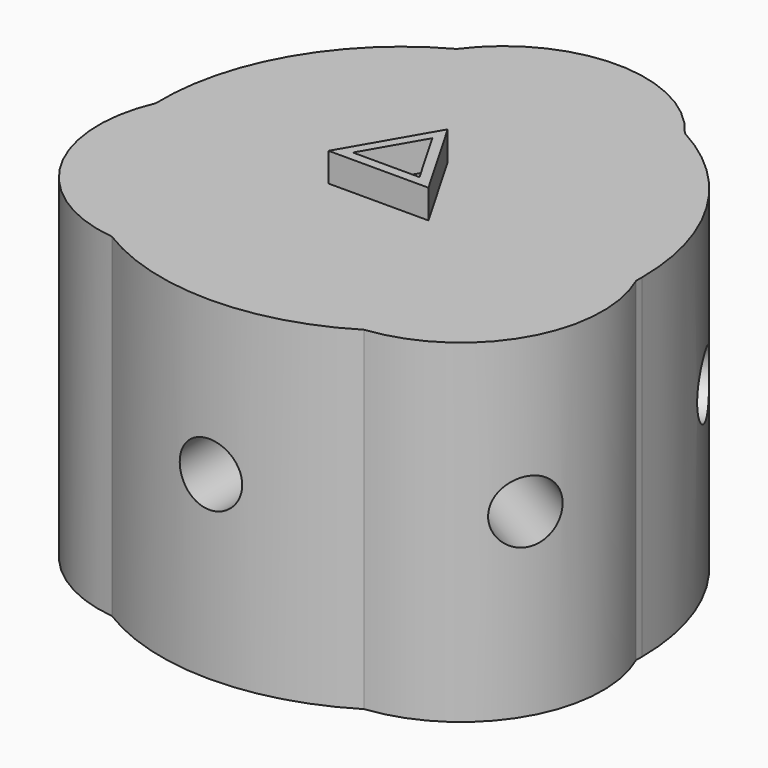
from build123d import *
from build123d import SkipClean  # not in build123d's __all__

# Parameters (mm, degrees)
F1_DEPTH       = 22
F3_R           = 3.25
F4_DEPTH       = 50
F4_DEPTH_BACK  = 50
F6_DEPTH       = 25
F7_R           = 3.25
F8_DEPTH       = 25
F8_DEPTH_BACK  = 40
F9_R           = 3.25
F10_DEPTH      = 25
F10_DEPTH_BACK = 40
F11_DEPTH      = 13.75
F13_DEPTH      = 250
F13_DEPTH_BACK = 250
F14_R          = 2.125
F15_DEPTH      = 100
F16_DEPTH      = 3


# Not quite as in the source:
# - after a boolean that leaves OpenCascade's solid faulty, fix() repairs it
# - a feature names something its author has since deleted; it is built from what else it names


with BuildPart() as f1:
    # F0 (on Top) → F1 (new body)
    with BuildSketch(Plane.XY):
        with BuildLine():
            ThreePointArc((-11.87, 22.002343057), (0, 25), (11.87, 22.002343057))
            ThreePointArc((11.87, 22.002343057), (0, 28), (-11.87, 22.002343057))
        make_face()
        with BuildLine():
            ThreePointArc((-13.1195880302, -21.2808930714), (-21.6506350946, -12.5), (-24.9895880302, -0.7214499856))
            ThreePointArc((-24.9895880302, -0.7214499856), (-24.248711306, -14), (-13.1195880302, -21.2808930714))
        make_face()
        with BuildLine():
            ThreePointArc((13.1195880302, -21.2808930714), (24.248711306, -14), (24.9895880302, -0.7214499856))
            ThreePointArc((24.9895880302, -0.7214499856), (21.6506350946, -12.5), (13.1195880302, -21.2808930714))
        make_face()
        with BuildLine():
            ThreePointArc((24.9895880302, -0.7214499856), (24.997396872, -0.3607625572), (25, 0))
            ThreePointArc((25, 0), (21.467999441, 12.8111279753), (11.87, 22.002343057))
            ThreePointArc((11.87, 22.002343057), (0, 25), (-11.87, 22.002343057))
            ThreePointArc((-11.87, 22.002343057), (-21.6506350946, 12.5), (-24.9895880302, -0.7214499856))
            ThreePointArc((-24.9895880302, -0.7214499856), (-21.6506350946, -12.5), (-13.1195880302, -21.2808930714))
            ThreePointArc((-13.1195880302, -21.2808930714), (0, -25), (13.1195880302, -21.2808930714))
            ThreePointArc((13.1195880302, -21.2808930714), (21.6506350946, -12.5), (24.9895880302, -0.7214499856))
        make_face()
    extrude(amount=F1_DEPTH)

    # F3 (on offset) → F4 (cut, two sides)
    with BuildSketch(Plane.XZ) as f4_sk:
        with Locations((0, 6)):
            Circle(F3_R)
    extrude(amount=F4_DEPTH, mode=Mode.SUBTRACT)
    extrude(f4_sk.sketch, amount=-F4_DEPTH_BACK, mode=Mode.SUBTRACT)

    # F7 (on face) → F8 (cut, two sides)
    with BuildSketch(Plane(origin=(-2.5980762114, 1.5, 0), x_dir=(-0.5, -0.8660254038, 0), z_dir=(-0.8660254038, 0.5, 0))) as f8_sk:
        with Locations((0, 6)):
            Circle(F7_R)
    extrude(amount=F8_DEPTH, mode=Mode.SUBTRACT)
    extrude(f8_sk.sketch, amount=-F8_DEPTH_BACK, mode=Mode.SUBTRACT)

    # F9 (on face) → F10 (cut, two sides)
    with BuildSketch(Plane(origin=(2.5980762114, 1.5, 0), x_dir=(-0.5, 0.8660254038, 0), z_dir=(0.8660254038, 0.5, 0))) as f10_sk:
        with Locations((0, 6)):
            Circle(F9_R)
    extrude(amount=F10_DEPTH, mode=Mode.SUBTRACT)
    extrude(f10_sk.sketch, amount=-F10_DEPTH_BACK, mode=Mode.SUBTRACT)

    # F0 (on Top) → F11 (join)
    with BuildSketch(Plane.XY):
        with BuildLine():
            ThreePointArc((24.9895880302, -0.7214499856), (24.997396872, -0.3607625572), (25, 0))
            ThreePointArc((25, 0), (21.467999441, 12.8111279753), (11.87, 22.002343057))
            ThreePointArc((11.87, 22.002343057), (0, 25), (-11.87, 22.002343057))
            ThreePointArc((-11.87, 22.002343057), (-21.6506350946, 12.5), (-24.9895880302, -0.7214499856))
            ThreePointArc((-24.9895880302, -0.7214499856), (-21.6506350946, -12.5), (-13.1195880302, -21.2808930714))
            ThreePointArc((-13.1195880302, -21.2808930714), (0, -25), (13.1195880302, -21.2808930714))
            ThreePointArc((13.1195880302, -21.2808930714), (21.6506350946, -12.5), (24.9895880302, -0.7214499856))
        make_face()
        with BuildLine():
            ThreePointArc((-11.87, 22.002343057), (0, 25), (11.87, 22.002343057))
            ThreePointArc((11.87, 22.002343057), (0, 28), (-11.87, 22.002343057))
        make_face()
        with BuildLine():
            ThreePointArc((13.1195880302, -21.2808930714), (24.248711306, -14), (24.9895880302, -0.7214499856))
            ThreePointArc((24.9895880302, -0.7214499856), (21.6506350946, -12.5), (13.1195880302, -21.2808930714))
        make_face()
        with BuildLine():
            ThreePointArc((-13.1195880302, -21.2808930714), (-21.6506350946, -12.5), (-24.9895880302, -0.7214499856))
            ThreePointArc((-24.9895880302, -0.7214499856), (-24.248711306, -14), (-13.1195880302, -21.2808930714))
        make_face()
    with SkipClean():  # cleaning this boolean's faces spoils the solid; the shape is the same uncleaned
        extrude(amount=-F11_DEPTH)

    # F12 (on Front) → F13 (cut, two sides)
    with BuildSketch(Plane.XZ) as f13_sk:
        Polygon((-63.1195880302, -13.75), (-13.1195880302, -13.75), (13.1195880302, -13.75), (63.1195880302, -13.75), (63.1195880302, -12.75), (0, -12.75), (-63.1195880302, -12.75), align=None)
    extrude(amount=-F13_DEPTH, mode=Mode.SUBTRACT)
    extrude(f13_sk.sketch, amount=F13_DEPTH_BACK, mode=Mode.SUBTRACT)

    add(f1.part.fix(), mode=Mode.REPLACE)

    # F14 (on face) → F15 (cut)
    with BuildSketch(Plane(origin=(0, 0, -12.75), x_dir=(1, 0, 0), z_dir=(0, 0, -1))):
        Circle(F14_R)
    extrude(amount=-F15_DEPTH, mode=Mode.SUBTRACT)

    # F14 (on face) → F16 (cut)
    with BuildSketch(Plane(origin=(0, 0, -12.75), x_dir=(1, 0, 0), z_dir=(0, 0, -1))):
        Polygon((0.3890172707, -4.3126170202), (3.9293445317, -1.8194096711), (3.5403272609, 2.4932073491), (-0.3890172707, 4.3126170202), (-3.9293445317, 1.8194096711), (-3.5403272609, -2.4932073491), align=None)
        Circle(F14_R, mode=Mode.SUBTRACT)
    extrude(amount=-F16_DEPTH, mode=Mode.SUBTRACT)


with BuildPart() as f6:
    # F5 (on Top) → F6 (new body)
    with BuildSketch(Plane.XY):
        Polygon((-5.1961524227, -3), (5.1961524227, -3), (0, 6), align=None)
        Polygon((0, 4), (3.4641016151, -2), (-3.4641016151, -2), align=None, mode=Mode.SUBTRACT)
    extrude(amount=F6_DEPTH)


solid = Compound([f1.part, f6.part])
